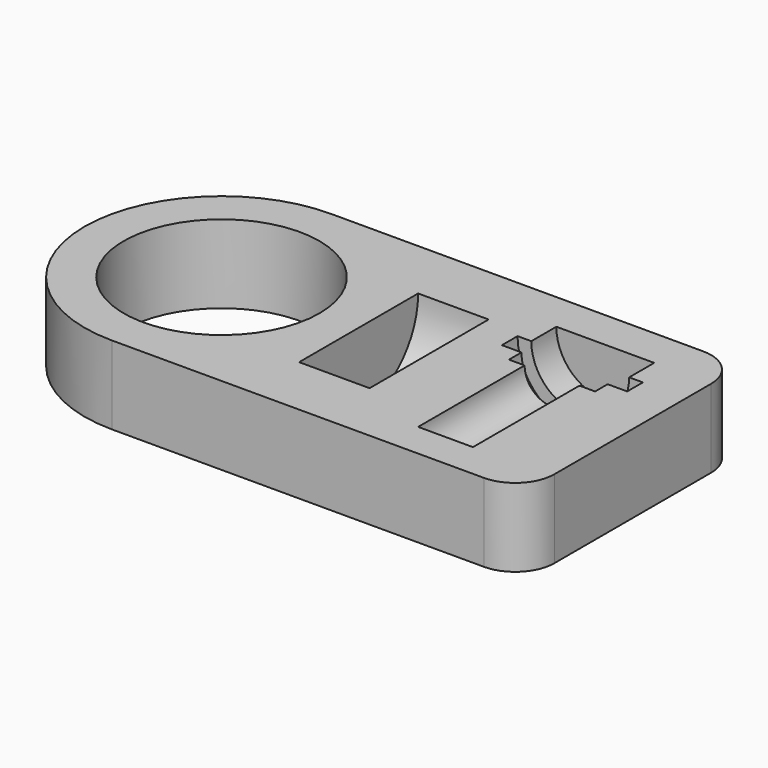
from build123d import *

# Parameters (mm, degrees)
F0_R         = 12.5
F1_DEPTH     = 10
F2_W         = 9
F2_H         = 9.5
F5_TEXT_SIZE = 5.5555555556
F6_DEPTH     = 1


# Not quite as in the source:
# - Text() gives the source's letters only with a copy of the font that has no kerning and outlines rounded to 1/6400 em; it was checked with that copy


with BuildPart() as f1:
    # F0 (on Top) → F1 (new body)
    with BuildSketch(Plane.XY):
        with BuildLine():
            ThreePointArc((0, 17.5), (5.1256313292, 5.1256313292), (17.5, 0))
            Line((17.5, 0), (65, 0))
            ThreePointArc((65, 0), (68.5355339059, 1.4644660941), (70, 5))
            Line((70, 5), (70, 30))
            ThreePointArc((70, 30), (68.5355339059, 33.5355339059), (65, 35))
            Line((65, 35), (17.5, 35))
            ThreePointArc((17.5, 35), (5.1256313292, 29.8743686708), (0, 17.5))
        make_face()
        with Locations((17.5, 17.5)):
            Circle(F0_R, mode=Mode.SUBTRACT)
    extrude(amount=F1_DEPTH)

    # F2 (on face) → F3 (revolve, cut)
    with BuildSketch(Plane.XY.offset(10)):
        with Locations((39.5, 12.75)):
            Rectangle(F2_W, F2_H)
    revolve(axis=Axis((39.5, 17.5, 10), (1, 0, 0)), mode=Mode.SUBTRACT)

    # F2 (on face) → F4 (revolve, cut)
    with BuildSketch(Plane.XY.offset(10)):
        Polygon((62.75, 30), (56.5, 30), (56.5, 26), (56.5, 23.5), (56.5, 21.5), (56.5, 4.5), (60, 4.5), (60, 21.5), (62, 21.5), (62, 23.5), (64.5, 23.5), (64.5, 26), (62.75, 26), align=None)
    revolve(axis=Axis((56.5, 13, 10), (0, -1, 0)), mode=Mode.SUBTRACT)

    # F5 (on face) → F6 (cut)
    with BuildSketch(Plane(origin=(0, 0, 0), x_dir=(1, 0, 0), z_dir=(0, 0, -1))):
        with Locations((30, -9)):
            Text('916, 1018', F5_TEXT_SIZE, font='Open Sans', text_align=(TextAlign.LEFT, TextAlign.BOTTOM))
    extrude(amount=-F6_DEPTH, mode=Mode.SUBTRACT)


solid = f1.part
